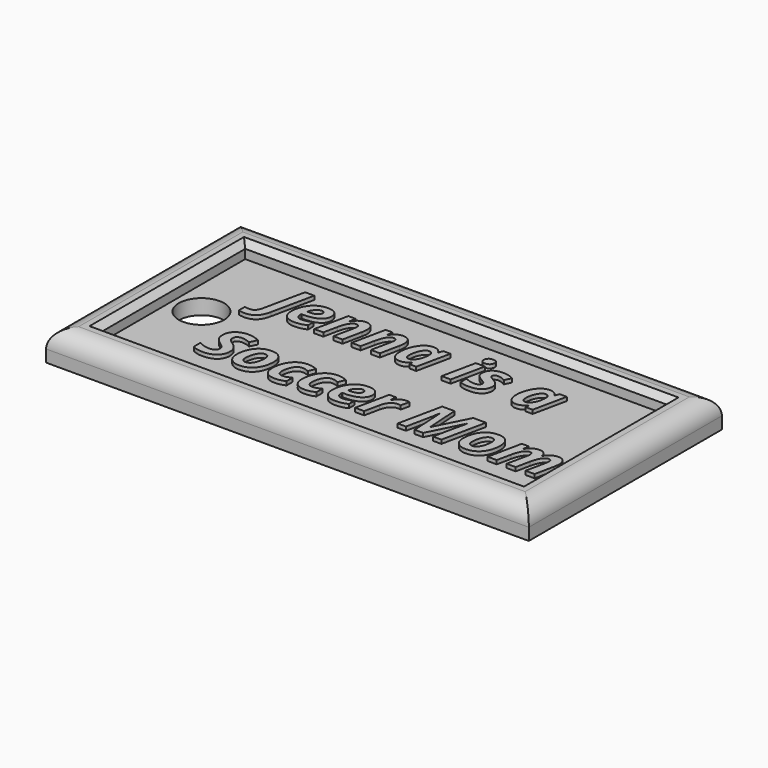
from build123d import *

# Parameters (mm, degrees)
F0_W         = 44.45
F0_H         = 19.05
F0_R         = 2.38125
F1_DEPTH     = 1.5875
F0_W_2       = 50.8
F0_H_2       = 25.4
F2_DEPTH     = 3.175
F3_R         = 1.905
F4_SIZE      = 0.635
F5_TEXT_SIZE = 6.5020532238
F6_DEPTH     = 0.396875


# Not quite as in the source:
# - Text() gives the source's letters only with a copy of the font that has no kerning and outlines rounded to 1/6400 em; it was checked with that copy


with BuildPart() as f1:
    # F0 (on Top) → F1 (new body)
    with BuildSketch(Plane.XY):
        with Locations((25.4, 12.7)):
            Rectangle(F0_W, F0_H)
        with Locations((6.19125, 12.7)):
            Circle(F0_R, mode=Mode.SUBTRACT)
    extrude(amount=F1_DEPTH)

    # F0 (on Top) → F2 (join)
    with BuildSketch(Plane.XY):
        with Locations((25.4, 12.7)):
            Rectangle(F0_W_2, F0_H_2)
        with Locations((25.4, 12.7)):
            Rectangle(F0_W, F0_H, mode=Mode.SUBTRACT)
    extrude(amount=F2_DEPTH)

    # F3
    f3_edges = [f1.edges().sort_by_distance(p)[0] for p in [
        (25.4, 0, 3.175),
        (50.8, 12.7, 3.175),
        (25.4, 25.4, 3.175),
        (0, 12.7, 3.175),
    ]]
    fillet(f3_edges, radius=F3_R)

    # F4
    f4_edges = [f1.edges().sort_by_distance(p)[0] for p in [
        (25.4, 22.225, 3.175),
        (3.175, 12.7, 3.175),
        (25.4, 3.175, 3.175),
        (47.625, 12.7, 3.175),
    ]]
    chamfer(f4_edges, length=F4_SIZE)

    # F5 (on face) → F6 (join)
    with BuildSketch(Plane.XY.offset(1.5875)):
        with Locations((9.955119333, 15.4583068941)):
            Text('Jenna is a', F5_TEXT_SIZE, font='Open Sans', font_style=FontStyle.BOLDITALIC, text_align=(TextAlign.LEFT, TextAlign.BOTTOM))
        with Locations((9.955119333, 6.6155145097)):
            Text('Soccer Mom', F5_TEXT_SIZE, font='Open Sans', font_style=FontStyle.BOLDITALIC, text_align=(TextAlign.LEFT, TextAlign.BOTTOM))
    extrude(amount=F6_DEPTH)


solid = f1.part
